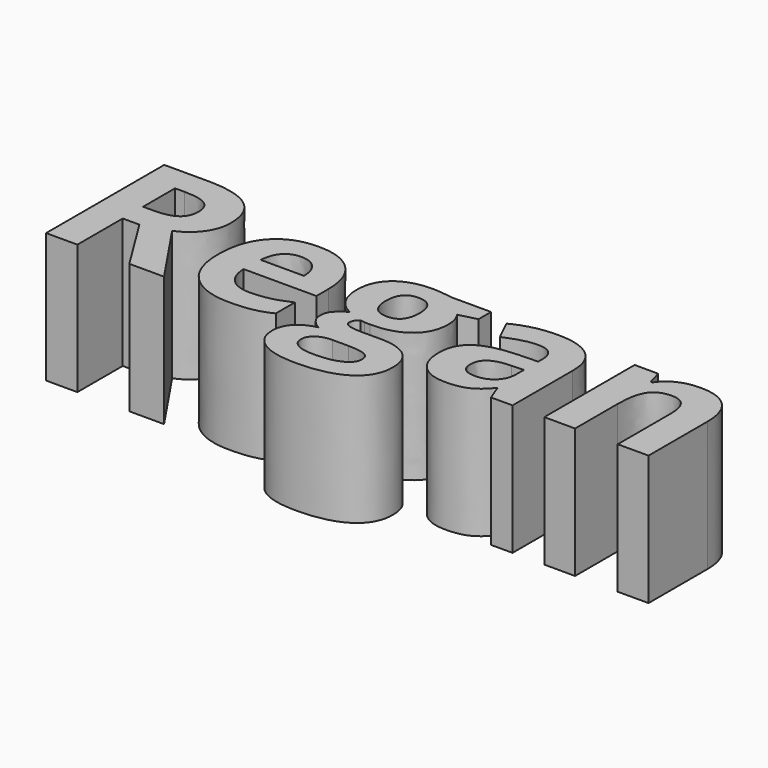
from build123d import *

# Parameters (mm, degrees)
F0_TEXT_SIZE = 148.5074508107
F1_DEPTH     = 93.218


# Not quite as in the source:
# - Text() gives the source's letters only with a copy of the font that has no kerning and outlines rounded to 1/6400 em; it was checked with that copy


with BuildPart() as f1:
    # F0 (on Top) → F1 (new body)
    with BuildSketch(Plane.XY):
        with Locations((-142.2034054995, -52.6971966028)):
            Text('Regan', F0_TEXT_SIZE, font='Open Sans', font_style=FontStyle.BOLD, text_align=(TextAlign.LEFT, TextAlign.BOTTOM))
    extrude(amount=F1_DEPTH)


solid = f1.part
